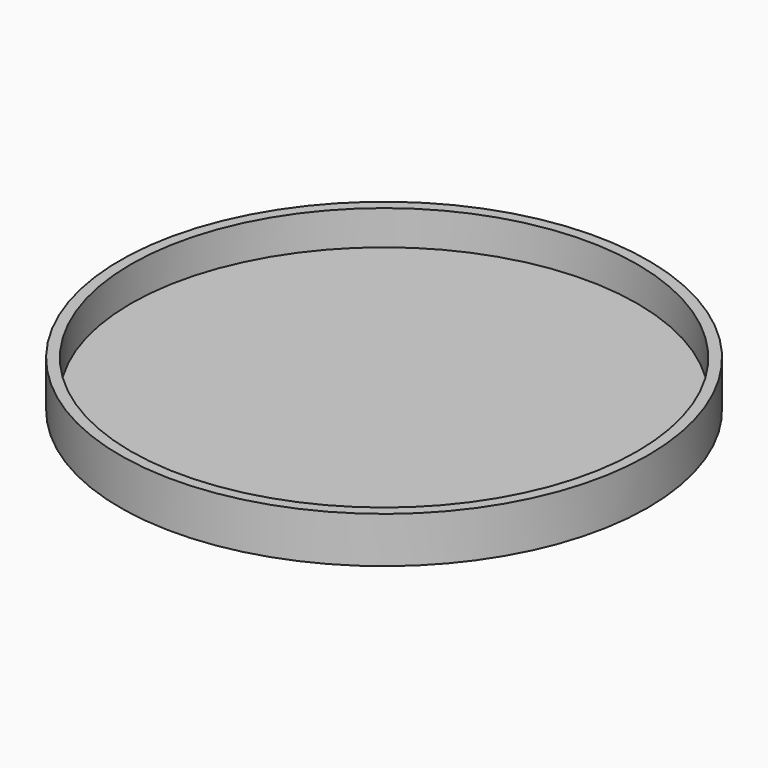
from build123d import *

# Parameters (mm, degrees)
F0_R     = 33.5
F1_DEPTH = 1.5
F2_R     = 34.4
F2_R_2   = 33
F3_DEPTH = 6


# Not quite as in the source:
# - the program builds the solid bodies; features that only make, move or delete a surface that nothing else refers to are left out


with BuildPart() as f1:
    # F0 (on Top) → F1 (new body)
    with BuildSketch(Plane.XY):
        Circle(F0_R)
    extrude(amount=F1_DEPTH)

    # F2 (on Top) → F3 (join)
    with BuildSketch(Plane.XY):
        Circle(F2_R)
        Circle(F2_R_2, mode=Mode.SUBTRACT)
    extrude(amount=F3_DEPTH)


solid = f1.part
